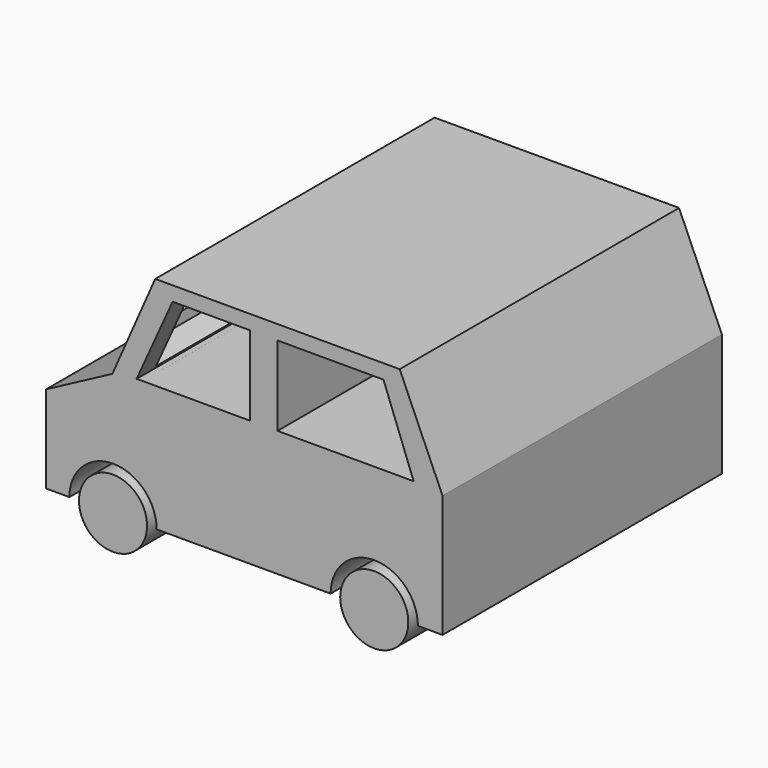
from build123d import *

# Parameters (mm, degrees)
F1_DEPTH         = 50.8
F3_DEPTH         = 7.62
F3_COPIES_COUNT  = 2
F3_COPIES_PITCH  = 43.180422
F3_COPIES1_COUNT = 2
F3_COPIES1_PITCH = 57.645984
F5_DEPTH         = 7.62
F7_DEPTH         = 7.62
F9_DEPTH         = 7.62
F11_DEPTH        = 76.2
F13_DEPTH        = 76.2
F14_W            = 45.0653012376
F14_H            = 10.795
F15_DEPTH        = 3.81
F17_DEPTH        = 7.62
F19_DEPTH        = 7.62
F21_DEPTH        = 7.62
F23_DEPTH        = 7.62


# Not quite as in the source:
# - a pattern or mirror of a feature is missing from the dataset's text; its kind, count and spacing are read off the source's solid


with BuildPart() as f1:
    # F0 (on Front) → F1 (new body)
    with BuildSketch(Plane.XZ):
        Polygon((-75.7135227323, 45.2577668846), (-75.7135227323, 32.5577668846), (-18.04306696, 32.5577668846), (-18.04306696, 34.4673171639), (-18.04306696, 50.3806362459), (-24.2752695117, 64.5659697758), (-59.8352695117, 64.5659697758), (-66.0674720634, 50.3806362459), align=None)
    extrude(amount=F1_DEPTH)

    # F2 (on face) → F3 (cut)
    with BuildSketch(Plane.XZ.offset(50.8)):
        with BuildLine():
            Line((-72.3248315811, 32.5577668846), (-59.6248315811, 32.5577668846))
            ThreePointArc((-59.6248315811, 32.5577668846), (-65.9748315811, 38.9077668846), (-72.3248315811, 32.5577668846))
        make_face()
    f3 = extrude(amount=-F3_DEPTH, mode=Mode.SUBTRACT)

    # F3_copies: F3 ×2
    with Locations(*[Vector(-0.004422337, 0.9999902214, 0) * (i * F3_COPIES_PITCH) for i in range(1, F3_COPIES_COUNT)]):
        add(f3, mode=Mode.SUBTRACT)

    # F3_copies1: F3 ×2
    with Locations(*[Vector(0.662508063, 0.749054782, 0) * (i * F3_COPIES1_PITCH) for i in range(1, F3_COPIES1_COUNT)]):
        add(f3, mode=Mode.SUBTRACT)

    # F4 (on face) → F5 (join)
    with BuildSketch(Plane.XZ.offset(43.18)):
        with BuildLine():
            Line((-70.9278315811, 32.5577668846), (-61.0218315811, 32.5577668846))
            ThreePointArc((-61.0218315811, 32.5577668846), (-65.9748315811, 37.5107668846), (-70.9278315811, 32.5577668846))
        make_face()
        with BuildLine():
            ThreePointArc((-70.9278315811, 32.5577668846), (-65.9748315811, 27.6047668846), (-61.0218315811, 32.5577668846))
            Line((-61.0218315811, 32.5577668846), (-70.9278315811, 32.5577668846))
        make_face()
    extrude(amount=F5_DEPTH)

    # F6 (on face) → F7 (cut)
    with BuildSketch(Plane.XZ.offset(50.8)):
        with BuildLine():
            Line((-34.3248570174, 32.5577668846), (-21.6248570174, 32.5577668846))
            ThreePointArc((-21.6248570174, 32.5577668846), (-27.9748570174, 38.9077668846), (-34.3248570174, 32.5577668846))
        make_face()
    extrude(amount=-F7_DEPTH, mode=Mode.SUBTRACT)

    # F8 (on face) → F9 (join)
    with BuildSketch(Plane.XZ.offset(43.18)):
        with BuildLine():
            Line((-32.9278570174, 32.5577668846), (-23.0218570174, 32.5577668846))
            ThreePointArc((-23.0218570174, 32.5577668846), (-27.9748570174, 37.5107668846), (-32.9278570174, 32.5577668846))
        make_face()
        with BuildLine():
            ThreePointArc((-32.9278570174, 32.5577668846), (-27.9748570174, 27.6047668846), (-23.0218570174, 32.5577668846))
            Line((-23.0218570174, 32.5577668846), (-32.9278570174, 32.5577668846))
        make_face()
    extrude(amount=F9_DEPTH)

    # F10 (on face) → F11 (cut)
    with BuildSketch(Plane.XZ.offset(50.8)):
        Polygon((-46.0276552343, 62.4638214125), (-57.3104978095, 62.4638214125), (-62.5376552343, 50.8894175291), (-46.0276552343, 50.8894175291), align=None)
    extrude(amount=-F11_DEPTH, mode=Mode.SUBTRACT)

    # F12 (on face) → F13 (cut)
    with BuildSketch(Plane.XZ.offset(50.8)):
        Polygon((-26.6381744295, 62.4638214125), (-42.0552695117, 62.4638214125), (-42.0552695117, 50.8814214125), (-22.2462173551, 50.8814214125), align=None)
    extrude(amount=-F13_DEPTH, mode=Mode.SUBTRACT)

    # F14 (on face) → F15 (cut)
    with BuildSketch(Plane(origin=(-73.9314589089, 0, 32.4811415881), x_dir=(0, -1, 0), z_dir=(-0.9155372099, 0, 0.4022332872))):
        with Locations((24.9195831129, 27.1725985175)):
            Rectangle(F14_W, F14_H)
    extrude(amount=-F15_DEPTH, mode=Mode.SUBTRACT)

    # F16 (on face) → F17 (cut)
    with BuildSketch(Plane(origin=(0, 0, 0), x_dir=(-1, 0, 0), z_dir=(0, 1, 0))):
        with BuildLine():
            ThreePointArc((21.433902362, 32.5577668846), (27.783902362, 26.2077668846), (34.133902362, 32.5577668846))
            ThreePointArc((34.133902362, 32.5577668846), (27.783902362, 38.9077668846), (21.433902362, 32.5577668846))
        make_face()
    extrude(amount=-F17_DEPTH, mode=Mode.SUBTRACT)

    # F18 (on face) → F19 (join)
    with BuildSketch(Plane(origin=(0, -7.62, 0), x_dir=(-1, 0, 0), z_dir=(0, 1, 0))):
        with BuildLine():
            Line((22.830902362, 32.5577668846), (32.736902362, 32.5577668846))
            ThreePointArc((32.736902362, 32.5577668846), (27.783902362, 37.5107668846), (22.830902362, 32.5577668846))
        make_face()
        with BuildLine():
            ThreePointArc((22.830902362, 32.5577668846), (27.783902362, 27.6047668846), (32.736902362, 32.5577668846))
            Line((32.736902362, 32.5577668846), (22.830902362, 32.5577668846))
        make_face()
    extrude(amount=F19_DEPTH)

    # F20 (on face) → F21 (cut)
    with BuildSketch(Plane(origin=(0, 0, 0), x_dir=(-1, 0, 0), z_dir=(0, 1, 0))):
        with BuildLine():
            ThreePointArc((59.8157899618, 32.5577668846), (66.1657899618, 26.2077668846), (72.5157899618, 32.5577668846))
            ThreePointArc((72.5157899618, 32.5577668846), (66.1657899618, 38.9077668846), (59.8157899618, 32.5577668846))
        make_face()
    extrude(amount=-F21_DEPTH, mode=Mode.SUBTRACT)

    # F22 (on face) → F23 (join)
    with BuildSketch(Plane(origin=(0, -7.62, 0), x_dir=(-1, 0, 0), z_dir=(0, 1, 0))):
        with BuildLine():
            ThreePointArc((61.2127899618, 32.5577668846), (66.1657899618, 27.6047668846), (71.1187899618, 32.5577668846))
            Line((71.1187899618, 32.5577668846), (61.2127899618, 32.5577668846))
        make_face()
        with BuildLine():
            Line((61.2127899618, 32.5577668846), (71.1187899618, 32.5577668846))
            ThreePointArc((71.1187899618, 32.5577668846), (66.1657899618, 37.5107668846), (61.2127899618, 32.5577668846))
        make_face()
    extrude(amount=F23_DEPTH)


solid = f1.part
